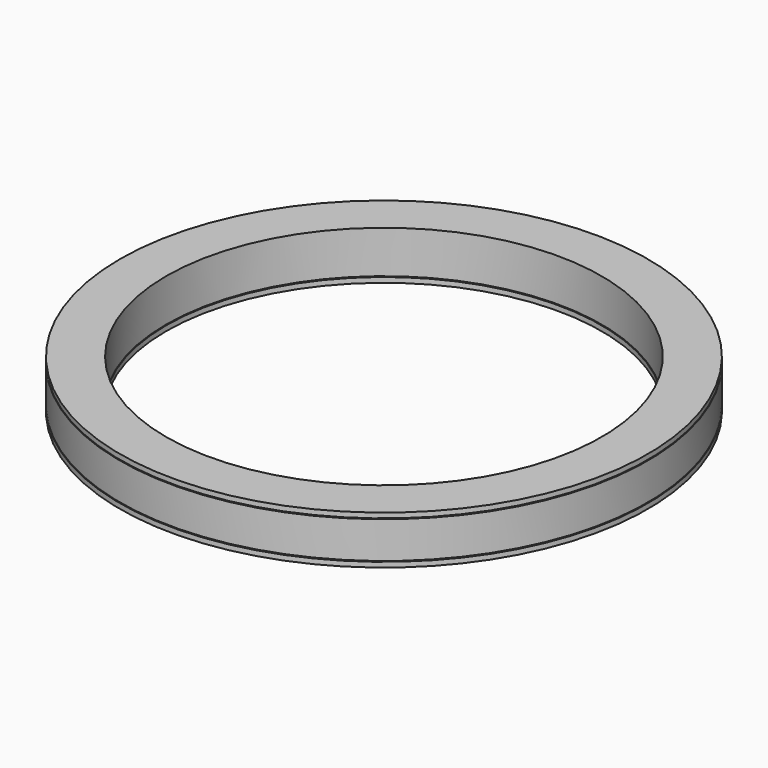
from build123d import *

# Parameters (mm, degrees)
F0_W            = 1.6
F0_H            = 3.6954253595
F3_DEPTH        = 7.9508945767
F3_COPIES_COUNT = 60
F0_H_2          = 11.6508945767


# Not quite as in the source:
# - ends of sketch curves that miss each other by under 0.0002 mm in the source are joined
# - a pattern or mirror of a feature is missing from the dataset's text; its kind, count and spacing are read off the source's solid
# - a feature names something its author has since deleted; it is built from what else it names


with BuildPart() as f1:
    # F0 (on Front) → F1 (revolve)
    with BuildSketch(Plane.XZ):
        with BuildLine():
            Line((-23.4322673833, 4.3690095041), (-23.4322673833, 8.0644348636))
            Line((-23.4322673833, 8.0644348636), (-23.4992546814, 8.0644348636))
            Line((-23.4992546814, 8.0644348636), (-24.7816277109, 8.8048132774))
            ThreePointArc((-24.7816277109, 8.8048132774), (-24.7881986574, 8.8086206944), (-24.7947789121, 8.8124119955))
            ThreePointArc((-24.7947789121, 8.8124119955), (-27.1645750375, 10.4087949547), (-29.2887299605, 12.3199040808))
            Line((-29.2887299605, 12.3199040808), (-32.7822673833, 12.3199040808))
            Line((-32.7822673833, 12.3199040808), (-32.7822673833, 4.3690095041))
            Line((-32.7822673833, 4.3690095041), (-32.1391644033, 4.3690095041))
            Line((-32.1391644033, 4.3690095041), (-30.0498791039, 5.5752589341))
            Line((-30.0498791039, 5.5752589341), (-30.0498791039, 4.3690095041))
            Line((-30.0498791039, 4.3690095041), (-23.4322673833, 4.3690095041))
        make_face()
        with Locations((-22.6322673833, 6.2167221839)):
            Rectangle(F0_W, F0_H)
        Polygon((-31.3921384513, 4.3690095041), (-30.0498791039, 4.3690095041), (-30.0498791039, 5.5752589341), (-32.1391644033, 4.3690095041), align=None)
    revolve(axis=Axis((49.0677326167, 0, 4.1288105428), (0, 0, -1)))

    # F2 (on face) → F3 (cut, through all)
    with BuildSketch(Plane.XY.offset(12.3199040808)):
        with BuildLine():
            Line((-34.4428691586, -3.1435954561), (-23.6822673833, -2.7385333666))
            Line((-23.6822673833, -2.7385333666), (-23.6307786944, -2.7365951743))
            ThreePointArc((-23.6307786944, -2.7365951743), (-23.6693940721, -1.368539754), (-23.6822673833, 0))
            ThreePointArc((-23.6822673833, 0), (-23.6665984275, 1.5098303063), (-23.6195983096, 3.0190102355))
            Line((-23.6195983096, 3.0190102355), (-34.4428691586, 3.4685461458))
            Line((-34.4428691586, 3.4685461458), (-34.4428691586, -3.1435954561))
        make_face()
    f3 = extrude(amount=-F3_DEPTH, mode=Mode.SUBTRACT)

    # F3_copies: F3 ×60 about axis
    f3_copies_axis = Axis((49.06773, 0, 0), (0, 0, 1))
    for i in range(1, F3_COPIES_COUNT):
        add(f3.rotate(f3_copies_axis, i * 360 / F3_COPIES_COUNT), mode=Mode.SUBTRACT)

    # F0 (on Front) → F4 (revolve)
    with BuildSketch(Plane.XZ):
        Polygon((-31.3921384513, 4.3690095041), (-30.0498791039, 4.3690095041), (-30.0498791039, 5.5752589341), (-32.1391644033, 4.3690095041), align=None)
    revolve(axis=Axis((49.0677326167, 0, 4.1288105428), (0, 0, -1)))


with BuildPart() as f5:
    # F0 (on Front) → F5 (revolve)
    with BuildSketch(Plane.XZ):
        Polygon((-19.9927523965, 1.6190095041), (-21.8322673833, 1.6190095041), (-21.8322673833, 0.0190095041), (-19.9927523965, 0), align=None)
        Polygon((-23.4322673833, 1.6190095041), (-31.1822673833, 1.6190095041), (-31.1822673833, 4.1190095041), (-32.580310714, 4.1190095041), (-32.7822673833, 4.0024097667), (-32.7822673833, 2.8190095041), (-32.7822673833, 1.6190095041), (-34.6322673833, 1.6190095041), (-34.6322673833, 0.0190095041), (-21.8322673833, 0.0190095041), (-21.8322673833, 1.6190095041), (-21.8322673833, 4.1190095041), (-23.4322673833, 4.1190095041), (-23.4322673833, 3.2372621942), align=None)
    revolve(axis=Axis((49.0677326167, 0, 4.1288105428), (0, 0, -1)))


with BuildPart() as f6:
    # F0 (on Front) → F6 (revolve)
    with BuildSketch(Plane.XZ):
        with BuildLine():
            Line((-23.4322673833, 8.3144348636), (-21.5822673833, 8.3144348636))
            Line((-21.5822673833, 8.3144348636), (-21.5822673833, 15.3699040808))
            Line((-21.5822673833, 15.3699040808), (-34.6322673833, 15.3699040808))
            Line((-34.6322673833, 15.3699040808), (-34.6322673833, 13.7699040808))
            Line((-34.6322673833, 13.7699040808), (-32.7822673833, 13.7699040808))
            Line((-32.7822673833, 13.7699040808), (-32.7822673833, 12.5699040808))
            Line((-32.7822673833, 12.5699040808), (-29.1822673833, 12.5699040808))
            ThreePointArc((-29.1822673833, 12.5699040808), (-29.061204598, 12.4443791569), (-28.9390626319, 12.3199040808))
            ThreePointArc((-28.9390626319, 12.3199040808), (-26.920400716, 10.5357620077), (-24.6822673833, 9.0361227001))
            Line((-24.6822673833, 9.0361227001), (-23.4322673833, 8.3144348636))
        make_face()
        Polygon((-21.5822673833, 8.0644348636), (-21.5822673833, 1.8690095041), (-19.9927523965, 1.8690095041), (-19.9927523965, 15.3699040808), (-21.5822673833, 15.3699040808), (-21.5822673833, 8.3144348636), align=None)
    revolve(axis=Axis((49.0677326167, 0, 4.1288105428), (0, 0, -1)))


with BuildPart() as f7:
    # F0 (on Front) → F7 (revolve)
    with BuildSketch(Plane.XZ):
        with Locations((-33.8322673833, 7.6944567924)):
            Rectangle(F0_W, F0_H_2)
    revolve(axis=Axis((49.0677326167, 0, 4.1288105428), (0, 0, -1)))


solid = Compound([f1.part, f5.part, f6.part, f7.part])
